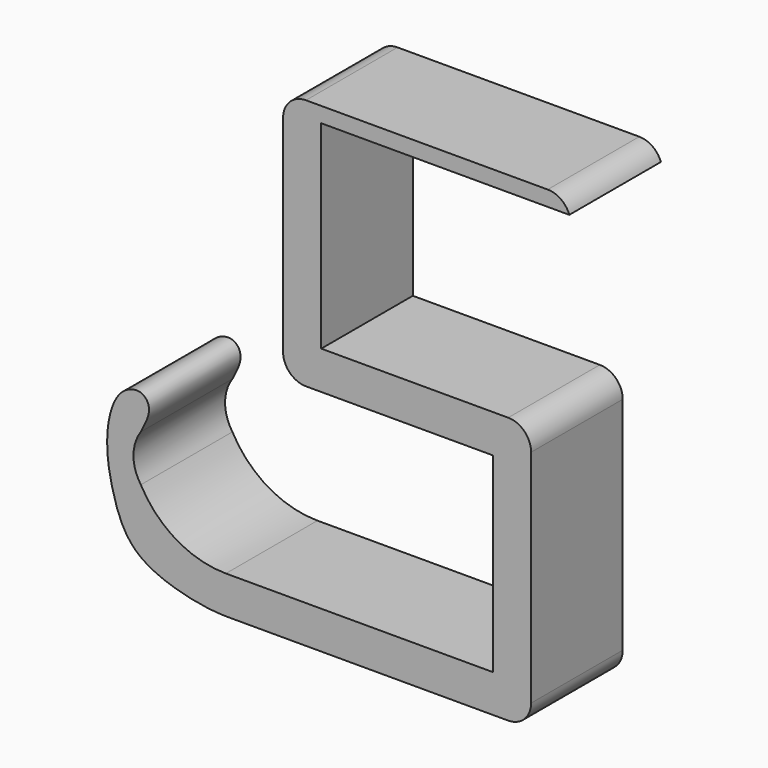
from build123d import *

# Parameters (mm, degrees)
F1_DEPTH    = 30
F2_T1_DEPTH = 60
F2_T3_DEPTH = 58.2842712475


# Not quite as in the source:
# - a fillet or chamfer that OpenCascade refuses, or shapes differently, is made with other operations: its cross-section is extruded or revolved along the edge and cut away or added


with BuildPart() as f1:
    # F0 (on Front) → F1 (new body)
    with BuildSketch(Plane.XZ):
        with BuildLine():
            Line((-20.4576485604, 41.7964319587), (44.5423514396, 41.7964319587))
            Line((44.5423514396, 41.7964319587), (44.5423514396, 45.7964319587))
            Line((44.5423514396, 45.7964319587), (-30.4576485604, 45.7964319587))
            Line((-30.4576485604, 45.7964319587), (-30.4576485604, -20.2035680413))
            Line((-30.4576485604, -20.2035680413), (24.5423514396, -20.2035680413))
            Line((24.5423514396, -20.2035680413), (24.5423514396, -70.2035680413))
            Line((24.5423514396, -70.2035680413), (-45.4576485604, -70.2035680413))
            ThreePointArc((-45.4576485604, -70.2035680413), (-58.4112677552, -66.6488561684), (-67.7362307906, -56.9804906845))
            ThreePointArc((-67.7362307906, -56.9804906845), (-69.6667608001, -50.8724953979), (-67.7362307906, -44.7645001113))
            add(Edge.make_bspline(
                [(-67.7362307906, -44.7645001113), (-66.6047282738, -42.6134626855), (-64.6275870644, -38.8548278844), (-67.5118728603, -34.7496923274), (-74.2171267591, -36.6728128022), (-77.5629423301, -48.422372807), (-75.1680740571, -62.4394566894), (-69.641186524, -75.442468141), (-51.6938526184, -79.943801044), (-46.7813036843, -80.045612986), (-44.8976382613, -80.0846517086)],
                knots=[0, 0, 0, 0, 0.1047159829, 0.1829764247, 0.2776975731, 0.4158396611, 0.5724266185, 0.7228497918, 0.8937296562, 1, 1, 1, 1], degree=3))
            Line((-44.8976382613, -80.0846517086), (34.5423514396, -80.0846517086))
            Line((34.5423514396, -80.0846517086), (34.5423514396, -10.2035680413))
            Line((34.5423514396, -10.2035680413), (-20.4576485604, -10.2035680413))
            Line((-20.4576485604, -10.2035680413), (-20.4576485604, 41.7964319587))
        make_face()
    extrude(amount=F1_DEPTH)

    # F2: fillet of radius 6 on 5 edges, made by hand

    # F2_s2 → F2_t1 (cut)
    with BuildSketch(Plane.XZ.offset(-15)):
        with BuildLine():
            ThreePointArc((-24.4576485604, 45.7964319587), (-28.7002892475, 44.0390726458), (-30.4576485604, 39.7964319587))
            Line((-30.4576485604, 39.7964319587), (-30.4576485604, 45.7964319587))
            Line((-30.4576485604, 45.7964319587), (-24.4576485604, 45.7964319587))
        make_face()
        with BuildLine():
            ThreePointArc((-30.4576485604, -14.2035680413), (-28.7002892475, -18.4462087284), (-24.4576485604, -20.2035680413))
            Line((-24.4576485604, -20.2035680413), (-30.4576485604, -20.2035680413))
            Line((-30.4576485604, -20.2035680413), (-30.4576485604, -14.2035680413))
        make_face()
        with BuildLine():
            ThreePointArc((34.5423514396, -16.2035680413), (32.7849921267, -11.9609273542), (28.5423514396, -10.2035680413))
            Line((28.5423514396, -10.2035680413), (34.5423514396, -10.2035680413))
            Line((34.5423514396, -10.2035680413), (34.5423514396, -16.2035680413))
        make_face()
        with BuildLine():
            ThreePointArc((28.5423514396, -80.0846517086), (32.7849921267, -78.3272923957), (34.5423514396, -74.0846517086))
            Line((34.5423514396, -74.0846517086), (34.5423514396, -80.0846517086))
            Line((34.5423514396, -80.0846517086), (28.5423514396, -80.0846517086))
        make_face()
    extrude(amount=F2_T1_DEPTH, mode=Mode.SUBTRACT)

    # F2_s4 → F2_t3 (cut)
    with BuildSketch(Plane.XZ.offset(-14.1421356237)):
        with BuildLine():
            ThreePointArc((44.5423514396, 41.7964319587), (42.3495988052, 44.6954114442), (38.8854971901, 45.7964319587))
            Line((38.8854971901, 45.7964319587), (44.5423514396, 45.7964319587))
            Line((44.5423514396, 45.7964319587), (44.5423514396, 41.7964319587))
        make_face()
    extrude(amount=F2_T3_DEPTH, mode=Mode.SUBTRACT)


solid = f1.part
